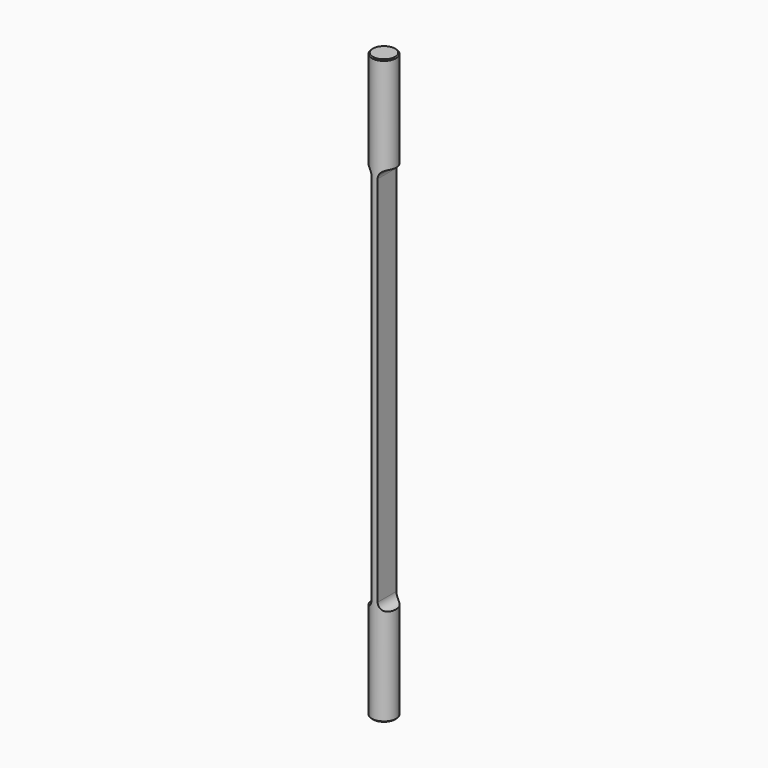
from build123d import *

# Parameters (mm, degrees)
F0_R     = 19.05
F1_DEPTH = 457.2
F2_SIZE2 = 1.5875
F2_SIZE  = 1.5875
F4_DEPTH = 19.05


# Not quite as in the source:
# - a pattern or mirror of a feature is missing from the dataset's text; its kind, count and spacing are read off the source's solid


with BuildPart() as f1:
    # F0 (on Top) → F1 (new body, symmetric)
    with BuildSketch(Plane.XY):
        Circle(F0_R)
    extrude(amount=F1_DEPTH, both=True)

    # F2
    f2_edges = [f1.edges().sort_by_distance(p)[0] for p in [
        (-19.05, 0, 457.2),
        (-19.05, 0, -457.2),
    ]]
    chamfer(f2_edges, length=F2_SIZE, length2=F2_SIZE2)

    # F3 (on Front) → F4 (cut, symmetric)
    with BuildSketch(Plane.XZ):
        with BuildLine():
            Line((4.7752, 292.1), (4.7752, -292.1))
            ThreePointArc((4.7752, -292.1), (17.4752, -304.8), (30.1752, -292.1))
            Line((30.1752, -292.1), (30.1752, 292.1))
            ThreePointArc((30.1752, 292.1), (17.4752, 304.8), (4.7752, 292.1))
        make_face()
    f4 = extrude(amount=F4_DEPTH, both=True, mode=Mode.SUBTRACT)

    # F4_copies: F4 across plane
    add(f4.mirror(Plane(origin=(0, 0, 0), x_dir=(0, 0, -1), z_dir=(-1, 0, 0))), mode=Mode.SUBTRACT)


solid = f1.part
